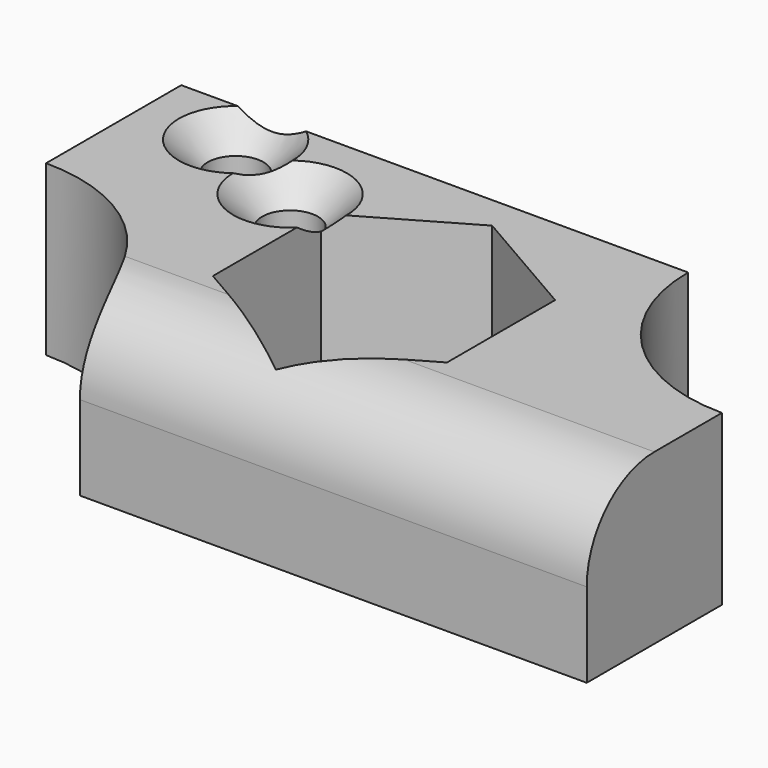
from build123d import *

# Parameters (mm, degrees)
F0_W           = 40
F0_H           = 20
F1_DEPTH       = 10
F3_DEPTH       = 25
F5_D           = 3.3
F5_CSINK_D     = 6.72
F5_CSINK_ANGLE = 90
F6_T1_DEPTH    = 55


# Not quite as in the source:
# - a fillet or chamfer that OpenCascade refuses, or shapes differently, is made with other operations: its cross-section is extruded or revolved along the edge and cut away or added


with BuildPart() as f1:
    # F0 (on Top) → F1 (new body)
    with BuildSketch(Plane.XY):
        Rectangle(F0_W, F0_H)
    extrude(amount=F1_DEPTH)

    # F2 (on face) → F3 (cut)
    with BuildSketch(Plane.XY.offset(10)):
        Polygon((0, -8), (6.9282032303, -4), (6.9282032303, 4), (0, 8), (-6.9282032303, 4), (-6.9282032303, -4), align=None)
        with BuildLine():
            ThreePointArc((-10, -10), (-12.9289321881, -2.9289321881), (-20, 0))
            Line((-20, 0), (-20, -10))
            Line((-20, -10), (-10, -10))
        make_face()
        with BuildLine():
            Line((20, 10), (10, 10))
            ThreePointArc((10, 10), (12.9289321881, 2.9289321881), (20, 0))
            Line((20, 0), (20, 10))
        make_face()
    extrude(amount=-F3_DEPTH, mode=Mode.SUBTRACT)

    # F5 (through all)
    with Locations(Plane.XY.offset(10)):
        with Locations((-14.633436854, 7.316718427), (-9.266873708, 4.633436854)):
            CounterSinkHole(F5_D / 2, F5_CSINK_D / 2, counter_sink_angle=F5_CSINK_ANGLE)

    # F6: fillet of radius 5 on 1 edges, made by hand

    # F6_s2 → F6_t1 (cut)
    with BuildSketch(Plane.YZ.offset(-22.5)):
        with BuildLine():
            ThreePointArc((-10, 5), (-8.5355339059, 8.5355339059), (-5, 10))
            Line((-5, 10), (-10, 10))
            Line((-10, 10), (-10, 5))
        make_face()
    extrude(amount=F6_T1_DEPTH, mode=Mode.SUBTRACT)


solid = f1.part
